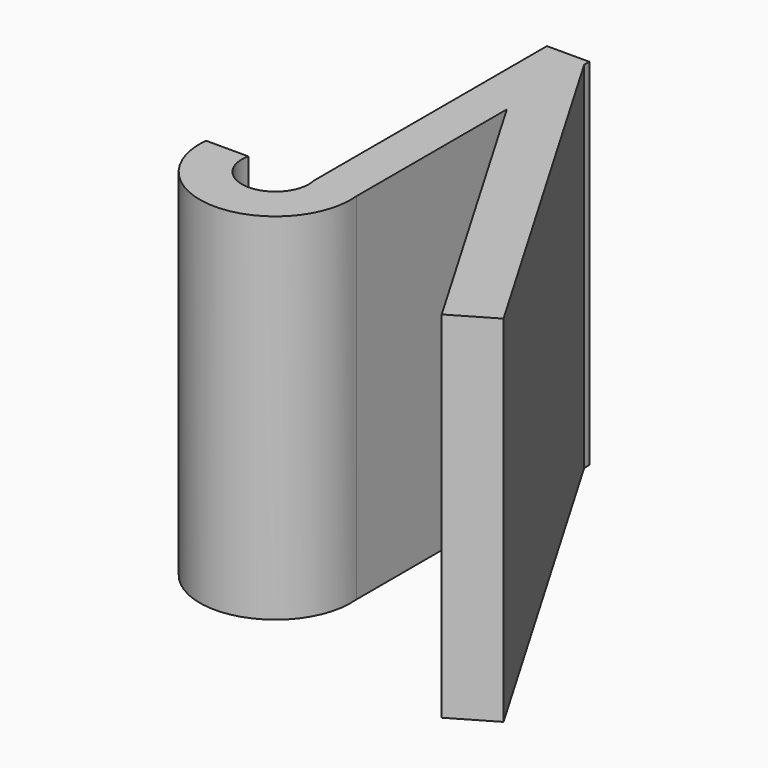
from build123d import *

# Parameters (mm, degrees)
F3_DEPTH = 42.3
F4_W     = 5.0520027294
F4_H     = 42.3
F5_DEPTH = 34.7
F7_DEPTH = 42.3


# Not quite as in the source:
# - the program builds the solid bodies; features that only make, move or delete a surface that nothing else refers to are left out


with BuildPart() as f3:
    # F0 (on Top) → F3 (new body)
    with BuildSketch(Plane.XY):
        with BuildLine():
            ThreePointArc((0, 0), (-3.9070909635, -4.8571115465), (-7.8141819269, 0))
            Line((-7.8141819269, 0), (-12.8661846563, 0))
            ThreePointArc((-12.8661846563, 0), (-3.9070909635, -9.8571115465), (5.0520027294, 0))
            Line((5.0520027294, 0), (0, 0))
        make_face()
    extrude(amount=F3_DEPTH)

    # F4 (on face) → F5 (join)
    with BuildSketch(Plane(origin=(0, 0, 0), x_dir=(-1, 0, 0), z_dir=(0, 1, 0))):
        with Locations((-2.5260013647, 21.15)):
            Rectangle(F4_W, F4_H)
    extrude(amount=F5_DEPTH)

    # F6 (on Top) → F7 (join)
    with BuildSketch(Plane.XY):
        Polygon((31.1498828232, -10.7009746134), (4.7412305139, 34.4645157456), (4.6712128018, 23.0707097992), (26.133000959, -13.6343887705), align=None)
    extrude(amount=F7_DEPTH)


solid = f3.part
